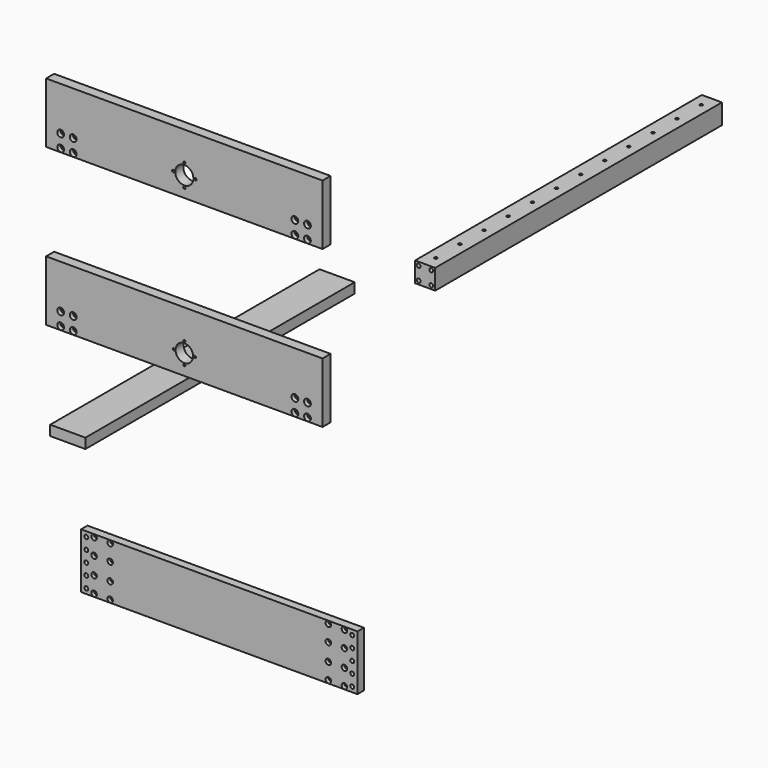
from build123d import *

# Parameters (mm, degrees)
F0_W             = 550
F0_H             = 120
F0_R             = 2.25
F0_R_2           = 18
F1_DEPTH         = 20
F0_W_2           = 40
F0_H_2           = 40
F0_R_3           = 4
F2_DEPTH         = 713
F0_R_4           = 17.4
F3_DEPTH         = 20
F0_W_3           = 70
F0_H_3           = 20
F4_DEPTH         = 669.8
F0_H_4           = 110
F5_DEPTH         = 16
F7_D             = 4.2
F8_D             = 8
F8_CBORE_D       = 13.5
F8_CBORE_DEPTH   = 8
F8_2_D           = 8
F8_2_CBORE_D     = 13.5
F8_2_CBORE_DEPTH = 8
F9_D             = 7.6
F10_D            = 5.8
F11_D            = 5.5
F11_CBORE_D      = 11
F11_CBORE_DEPTH  = 7
F12_D            = 7.8


# Not quite as in the source:
# - a feature names something its author has since deleted; it is built from what else it names


with BuildPart() as f1:
    # F0 (on Front) → F1 (new body)
    with BuildSketch(Plane.XZ):
        with Locations((-775.5616648197, 286.5064552142)):
            Rectangle(F0_W, F0_H)
        with Locations((-775.5616648197, 244.5064552142)):
            Circle(F0_R, mode=Mode.SUBTRACT)
        with Locations((-797.5616648197, 266.5064552142)):
            Circle(F0_R, mode=Mode.SUBTRACT)
        with Locations((-775.5616648197, 266.5064552142)):
            Circle(F0_R_2, mode=Mode.SUBTRACT)
        with Locations((-775.5616648197, 288.5064552142)):
            Circle(F0_R, mode=Mode.SUBTRACT)
        with Locations((-753.5616648197, 266.5064552142)):
            Circle(F0_R, mode=Mode.SUBTRACT)
    extrude(amount=-F1_DEPTH)

    # F8 (through all)
    with Locations(Plane.XZ):
        with Locations((-1021.5616648197, 259.5064552142), (-996.5616648197, 259.5064552142), (-996.5616648197, 233.5064552142), (-1021.5616648197, 233.5064552142), (-555.5616648197, 259.5064552142), (-555.5616648197, 233.5064552142), (-530.5616648197, 233.5064552142), (-530.5616648197, 259.5064552142), (-1021.5616648197, -52.1013047353), (-996.5616648197, -52.1013047353), (-996.5616648197, -78.1013047353), (-1021.5616648197, -78.1013047353), (-555.5616648197, -52.1013047353), (-530.5616648197, -52.1013047353), (-530.5616648197, -78.1013047353), (-555.5616648197, -78.1013047353)):
            CounterBoreHole(F8_D / 2, F8_CBORE_D / 2, F8_CBORE_DEPTH)


with BuildPart() as f2:
    # F0 (on Front) → F2 (new body)
    with BuildSketch(Plane.XZ):
        with Locations((-296.3649737835, 246.5064552142)):
            Rectangle(F0_W_2, F0_H_2)
        with Locations((-309.3649737835, 233.5064552142)):
            Circle(F0_R_3, mode=Mode.SUBTRACT)
        with Locations((-284.3649737835, 233.5064552142)):
            Circle(F0_R_3, mode=Mode.SUBTRACT)
        with Locations((-309.3649737835, 259.5064552142)):
            Circle(F0_R_3, mode=Mode.SUBTRACT)
        with Locations((-284.3649737835, 259.5064552142)):
            Circle(F0_R_3, mode=Mode.SUBTRACT)
        with Locations((-309.3649737835, 259.5064552142)):
            Circle(F0_R_3)
        with Locations((-309.3649737835, 233.5064552142)):
            Circle(F0_R_3)
        with Locations((-284.3649737835, 259.5064552142)):
            Circle(F0_R_3)
        with Locations((-284.3649737835, 233.5064552142)):
            Circle(F0_R_3)
    extrude(amount=-F2_DEPTH)

    # F9 (through all)
    with Locations(Plane.XZ):
        with Locations((-309.3649737835, 233.5064552142), (-309.3649737835, 259.5064552142), (-284.3649737835, 259.5064552142), (-284.3649737835, 233.5064552142)):
            Hole(F9_D / 2)

    # F10 (through all)
    with Locations(Plane.XY.offset(266.5064552142)):
        with Locations((-296.3649737835, 26.5), (-296.3649737835, 86.5), (-296.3649737835, 146.5), (-296.3649737835, 206.5), (-296.3649737835, 266.5), (-296.3649737835, 326.5), (-296.3649737835, 386.5), (-296.3649737835, 446.5), (-296.3649737835, 506.5), (-296.3649737835, 566.5), (-296.3649737835, 626.5), (-296.3649737835, 26.5), (-296.3649737835, 86.5), (-296.3649737835, 146.5), (-296.3649737835, 206.5), (-296.3649737835, 266.5), (-296.3649737835, 326.5), (-296.3649737835, 386.5), (-296.3649737835, 446.5), (-296.3649737835, 506.5), (-296.3649737835, 566.5), (-296.3649737835, 626.5), (-296.3649737835, 686.5)):
            Hole(F10_D / 2)


with BuildPart() as f3:
    # F0 (on Front) → F3 (new body)
    with BuildSketch(Plane.XZ):
        with Locations((-775.5616648197, -25.1013047353)):
            Rectangle(F0_W, F0_H)
        with Locations((-775.5616648197, -45.1013047353)):
            Circle(F0_R_4, mode=Mode.SUBTRACT)
    extrude(amount=-F3_DEPTH)

    # F7 (through all)
    with Locations(Plane.XZ):
        with Locations((-796.5616648197, -45.1013047353), (-775.5616648197, -24.1013047353), (-754.5616648197, -45.1013047353), (-775.5616648197, -66.1013047353)):
            Hole(F7_D / 2)

    # F8#2 (through all)
    with Locations(Plane.XZ):
        with Locations((-1021.5616648197, 259.5064552142), (-996.5616648197, 259.5064552142), (-996.5616648197, 233.5064552142), (-1021.5616648197, 233.5064552142), (-555.5616648197, 259.5064552142), (-555.5616648197, 233.5064552142), (-530.5616648197, 233.5064552142), (-530.5616648197, 259.5064552142), (-1021.5616648197, -52.1013047353), (-996.5616648197, -52.1013047353), (-996.5616648197, -78.1013047353), (-1021.5616648197, -78.1013047353), (-555.5616648197, -52.1013047353), (-530.5616648197, -52.1013047353), (-530.5616648197, -78.1013047353), (-555.5616648197, -78.1013047353)):
            CounterBoreHole(F8_2_D / 2, F8_2_CBORE_D / 2, F8_2_CBORE_DEPTH)


with BuildPart() as f4:
    # F0 (on Front) → F4 (new body)
    with BuildSketch(Plane.XZ):
        with Locations((-1007.3494577408, -267.2632241249)):
            Rectangle(F0_W_3, F0_H_3)
    extrude(amount=-F4_DEPTH)


with BuildPart() as f5:
    # F0 (on Front) → F5 (new body)
    with BuildSketch(Plane.XZ):
        with Locations((-706.0369319916, -475.5515027046)):
            Rectangle(F0_W, F0_H_4)
    extrude(amount=-F5_DEPTH)

    # F11 (through all)
    with Locations(Plane.XZ):
        with Locations((-955.0369319916, -458.3015027046), (-955.0369319916, -426.3015027046), (-923.0369319916, -426.3015027046), (-923.0369319916, -458.3015027046), (-923.0369319916, -492.8015027046), (-923.0369319916, -524.8015027046), (-955.0369319916, -492.8015027046), (-955.0369319916, -524.8015027046), (-489.0369319916, -426.3015027046), (-489.0369319916, -458.3015027046), (-489.0369319916, -492.8015027046), (-489.0369319916, -524.8015027046), (-457.0369319916, -524.8015027046), (-457.0369319916, -492.8015027046), (-457.0369319916, -458.3015027046), (-457.0369319916, -426.3015027046)):
            CounterBoreHole(F11_D / 2, F11_CBORE_D / 2, F11_CBORE_DEPTH)

    # F12 (through all)
    with Locations(Plane.XZ):
        with Locations((-970.5369319916, -430.5515027046), (-970.5369319916, -453.0515027046), (-970.5369319916, -475.5515027046), (-970.5369319916, -498.0515027046), (-970.5369319916, -520.5515027046), (-441.5369319916, -520.5515027046), (-441.5369319916, -498.0515027046), (-441.5369319916, -475.5515027046), (-441.5369319916, -453.0515027046), (-441.5369319916, -430.5515027046)):
            Hole(F12_D / 2)


solid = Compound([f1.part, f2.part, f3.part, f4.part, f5.part])
